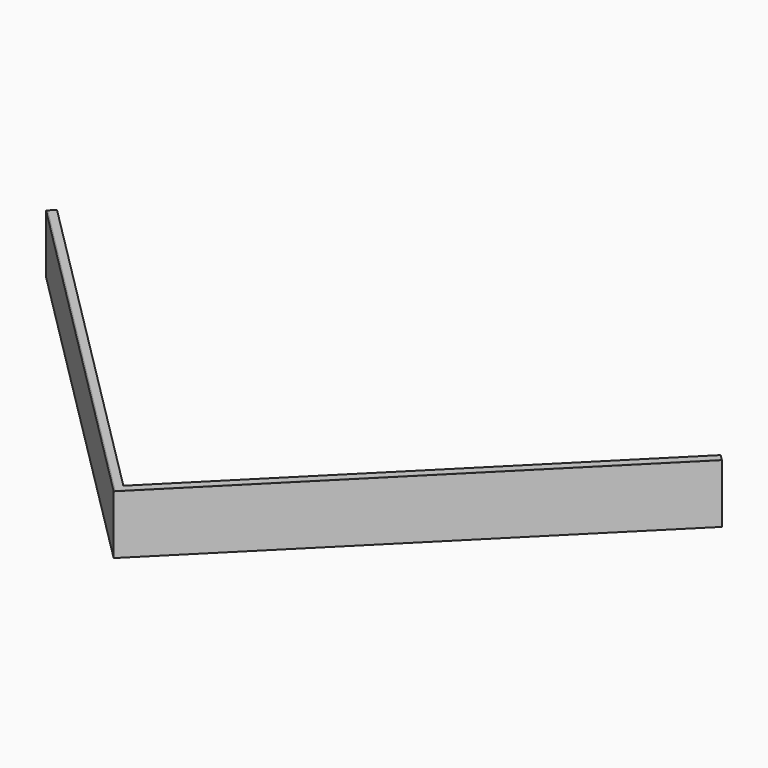
from build123d import *

# Parameters (mm, degrees)
F1_DEPTH = 304.8
F3_DEPTH = 6.35
F4_W     = 2433.6375
F4_H     = 31.75
F5_DEPTH = 6.35
F7_DEPTH = 6.35


with BuildPart() as f1:
    # F0 (on Top) → F1 (new body)
    with BuildSketch(Plane.XY):
        Polygon((-1752.2724756236, 1752.2724756236), (0, 0), (1752.2724756236, 1752.2724756236), (1747.7823475631, 1756.7626036842), (0, 8.9802561211), (-1747.7823475631, 1756.7626036842), align=None)
    extrude(amount=F1_DEPTH)


with BuildPart() as f3:
    # F2 (on face) → F3 (new body)
    with BuildSketch(Plane.XY.offset(304.8)):
        Polygon((-1720.8415791999, 1783.7033720474), (-1747.7823475631, 1756.7626036842), (0, 8.9802561211), (1747.7823475631, 1756.7626036842), (1720.8415791999, 1783.7033720474), (0, 62.8617928475), align=None)
    extrude(amount=-F3_DEPTH)

    # F6 (on face) → F7 (join)
    with BuildSketch(Plane(origin=(31.4308964237, 31.4308964237, 0), x_dir=(-0.7071067812, 0.7071067812, 0), z_dir=(0.7071067812, 0.7071067812, 0))):
        Polygon((2478.0875, 266.7), (2478.0875, 298.45), (44.45, 298.45), (44.4866344333, 266.7), align=None)
    extrude(amount=-F7_DEPTH)


with BuildPart() as f5:
    # F4 (on face) → F5 (new body)
    with BuildSketch(Plane(origin=(-31.4308964237, 31.4308964237, 0), x_dir=(-0.7071067812, -0.7071067812, 0), z_dir=(-0.7071067812, 0.7071067812, 0))):
        with Locations((-1261.26875, 282.575)):
            Rectangle(F4_W, F4_H)
    extrude(amount=-F5_DEPTH)


solid = Compound([f1.part, f3.part, f5.part])
